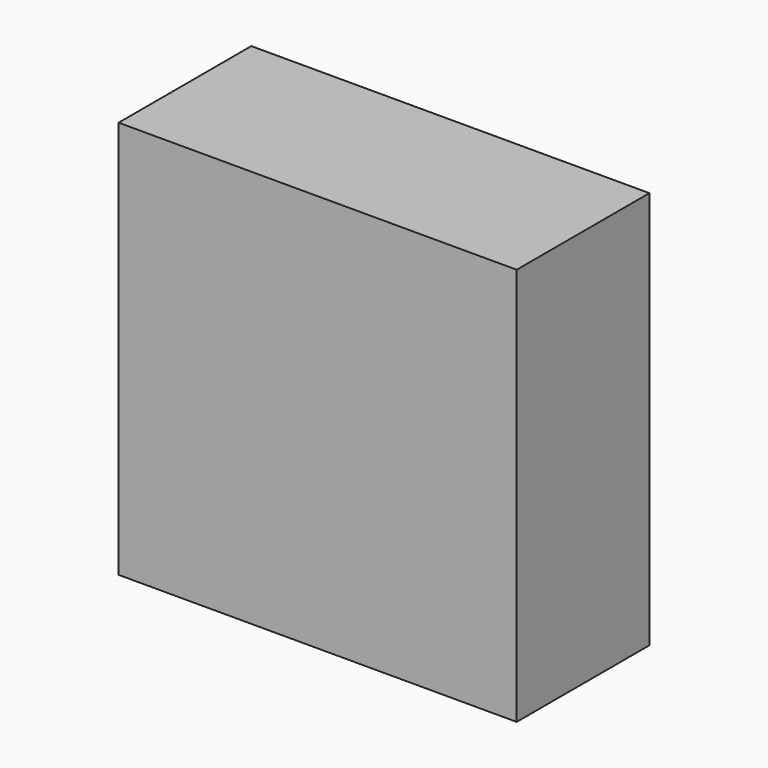
from build123d import *

# Parameters (mm, degrees)
F0_W     = 60
F0_H     = 60
F1_DEPTH = 25


# Not quite as in the source:
# - the program builds the solid bodies; features that only make, move or delete a surface that nothing else refers to are left out


with BuildPart() as f1:
    # F0 (on Front) → F1 (new body)
    with BuildSketch(Plane.XZ):
        with Locations((1.1512227356, -11.8655072413)):
            Rectangle(F0_W, F0_H)
    extrude(amount=F1_DEPTH)


solid = f1.part
